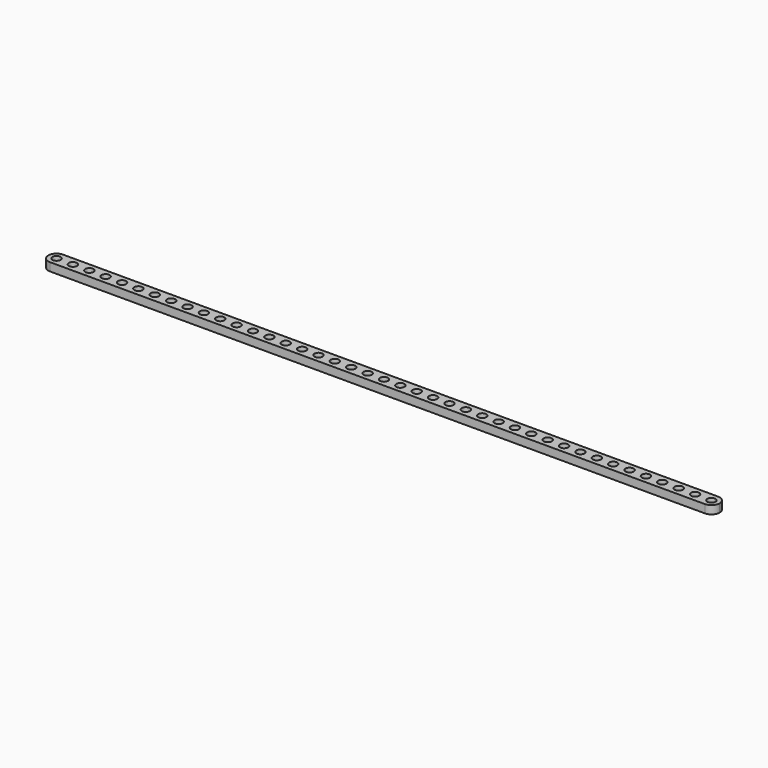
from build123d import *

# Parameters (mm, degrees)
F0_W      = 8
F0_H      = 4
F1_DEPTH  = 16
F2_DEPTH  = 24
F3_DEPTH  = 32
F4_DEPTH  = 40
F5_DEPTH  = 48
F6_DEPTH  = 56
F7_DEPTH  = 64
F8_DEPTH  = 72
F9_DEPTH  = 80
F10_DEPTH = 88
F11_DEPTH = 96
F12_DEPTH = 104
F13_DEPTH = 120
F14_DEPTH = 136
F15_DEPTH = 152
F16_DEPTH = 168
F17_DEPTH = 184
F18_DEPTH = 232
F19_DEPTH = 280
F20_DEPTH = 328
F21_R     = 2
F22_DEPTH = 12.5
F23_R     = 3.99999
F23_2_R   = 3.99999
F23_3_R   = 3.99999
F23_4_R   = 3.99999
F23_5_R   = 3.99999
F23_6_R   = 3.99999
F23_7_R   = 3.99999
F23_8_R   = 3.99999
F23_9_R   = 3.99999
F23_10_R  = 3.99999
F23_11_R  = 3.99999
F23_12_R  = 3.99999
F23_13_R  = 3.99999
F23_14_R  = 3.99999
F23_15_R  = 3.99999
F23_16_R  = 3.99999
F23_17_R  = 3.99999
F23_18_R  = 3.99999
F23_19_R  = 3.99999
F23_20_R  = 3.99999


# Not quite as in the source:
# - a fillet or chamfer is up to 0.001 mm smaller than in the source, because OpenCascade refuses the exact size


with BuildPart() as f1:
    # F0 (on Right) → F1 (new body)
    with BuildSketch(Plane.YZ):
        Rectangle(F0_W, F0_H)
    extrude(amount=F1_DEPTH)


with BuildPart() as f2:
    # F0 (on Right) → F2 (new body)
    with BuildSketch(Plane.YZ):
        Rectangle(F0_W, F0_H)
    extrude(amount=F2_DEPTH)


with BuildPart() as f3:
    # F0 (on Right) → F3 (new body)
    with BuildSketch(Plane.YZ):
        Rectangle(F0_W, F0_H)
    extrude(amount=F3_DEPTH)


with BuildPart() as f4:
    # F0 (on Right) → F4 (new body)
    with BuildSketch(Plane.YZ):
        Rectangle(F0_W, F0_H)
    extrude(amount=F4_DEPTH)


with BuildPart() as f5:
    # F0 (on Right) → F5 (new body)
    with BuildSketch(Plane.YZ):
        Rectangle(F0_W, F0_H)
    extrude(amount=F5_DEPTH)


with BuildPart() as f6:
    # F0 (on Right) → F6 (new body)
    with BuildSketch(Plane.YZ):
        Rectangle(F0_W, F0_H)
    extrude(amount=F6_DEPTH)


with BuildPart() as f7:
    # F0 (on Right) → F7 (new body)
    with BuildSketch(Plane.YZ):
        Rectangle(F0_W, F0_H)
    extrude(amount=F7_DEPTH)


with BuildPart() as f8:
    # F0 (on Right) → F8 (new body)
    with BuildSketch(Plane.YZ):
        Rectangle(F0_W, F0_H)
    extrude(amount=F8_DEPTH)


with BuildPart() as f9:
    # F0 (on Right) → F9 (new body)
    with BuildSketch(Plane.YZ):
        Rectangle(F0_W, F0_H)
    extrude(amount=F9_DEPTH)


with BuildPart() as f10:
    # F0 (on Right) → F10 (new body)
    with BuildSketch(Plane.YZ):
        Rectangle(F0_W, F0_H)
    extrude(amount=F10_DEPTH)


with BuildPart() as f11:
    # F0 (on Right) → F11 (new body)
    with BuildSketch(Plane.YZ):
        Rectangle(F0_W, F0_H)
    extrude(amount=F11_DEPTH)


with BuildPart() as f12:
    # F0 (on Right) → F12 (new body)
    with BuildSketch(Plane.YZ):
        Rectangle(F0_W, F0_H)
    extrude(amount=F12_DEPTH)


with BuildPart() as f13:
    # F0 (on Right) → F13 (new body)
    with BuildSketch(Plane.YZ):
        Rectangle(F0_W, F0_H)
    extrude(amount=F13_DEPTH)


with BuildPart() as f14:
    # F0 (on Right) → F14 (new body)
    with BuildSketch(Plane.YZ):
        Rectangle(F0_W, F0_H)
    extrude(amount=F14_DEPTH)


with BuildPart() as f15:
    # F0 (on Right) → F15 (new body)
    with BuildSketch(Plane.YZ):
        Rectangle(F0_W, F0_H)
    extrude(amount=F15_DEPTH)


with BuildPart() as f16:
    # F0 (on Right) → F16 (new body)
    with BuildSketch(Plane.YZ):
        Rectangle(F0_W, F0_H)
    extrude(amount=F16_DEPTH)


with BuildPart() as f17:
    # F0 (on Right) → F17 (new body)
    with BuildSketch(Plane.YZ):
        Rectangle(F0_W, F0_H)
    extrude(amount=F17_DEPTH)


with BuildPart() as f18:
    # F0 (on Right) → F18 (new body)
    with BuildSketch(Plane.YZ):
        Rectangle(F0_W, F0_H)
    extrude(amount=F18_DEPTH)


with BuildPart() as f19:
    # F0 (on Right) → F19 (new body)
    with BuildSketch(Plane.YZ):
        Rectangle(F0_W, F0_H)
    extrude(amount=F19_DEPTH)


with BuildPart() as f20:
    # F0 (on Right) → F20 (new body)
    with BuildSketch(Plane.YZ):
        Rectangle(F0_W, F0_H)
    extrude(amount=F20_DEPTH)


with BuildPart() as f22_tool:
    # F21 (on Top) → F22 (new body, symmetric)
    with BuildSketch(Plane.XY):
        with Locations((4, 0)):
            Circle(F21_R)
        with Locations((12, 0)):
            Circle(F21_R)
        with Locations((20, 0)):
            Circle(F21_R)
        with Locations((28, 0)):
            Circle(F21_R)
        with Locations((36, 0)):
            Circle(F21_R)
        with Locations((44, 0)):
            Circle(F21_R)
        with Locations((52, 0)):
            Circle(F21_R)
        with Locations((60, 0)):
            Circle(F21_R)
        with Locations((68, 0)):
            Circle(F21_R)
        with Locations((76, 0)):
            Circle(F21_R)
        with Locations((84, 0)):
            Circle(F21_R)
        with Locations((92, 0)):
            Circle(F21_R)
        with Locations((100, 0)):
            Circle(F21_R)
        with Locations((108, 0)):
            Circle(F21_R)
        with Locations((116, 0)):
            Circle(F21_R)
        with Locations((124, 0)):
            Circle(F21_R)
        with Locations((132, 0)):
            Circle(F21_R)
        with Locations((140, 0)):
            Circle(F21_R)
        with Locations((148, 0)):
            Circle(F21_R)
        with Locations((156, 0)):
            Circle(F21_R)
        with Locations((164, 0)):
            Circle(F21_R)
        with Locations((172, 0)):
            Circle(F21_R)
        with Locations((180, 0)):
            Circle(F21_R)
        with Locations((188, 0)):
            Circle(F21_R)
        with Locations((196, 0)):
            Circle(F21_R)
        with Locations((204, 0)):
            Circle(F21_R)
        with Locations((212, 0)):
            Circle(F21_R)
        with Locations((220, 0)):
            Circle(F21_R)
        with Locations((228, 0)):
            Circle(F21_R)
        with Locations((236, 0)):
            Circle(F21_R)
        with Locations((244, 0)):
            Circle(F21_R)
        with Locations((252, 0)):
            Circle(F21_R)
        with Locations((260, 0)):
            Circle(F21_R)
        with Locations((268, 0)):
            Circle(F21_R)
        with Locations((276, 0)):
            Circle(F21_R)
        with Locations((284, 0)):
            Circle(F21_R)
        with Locations((292, 0)):
            Circle(F21_R)
        with Locations((300, 0)):
            Circle(F21_R)
        with Locations((308, 0)):
            Circle(F21_R)
        with Locations((316, 0)):
            Circle(F21_R)
        with Locations((324, 0)):
            Circle(F21_R)
        with BuildLine():
            Line((4, 4), (0, 4))
            Line((0, 4), (0, 0))
            ThreePointArc((0, 0), (1.1715728753, 2.8284271247), (4, 4))
        make_face()
        with BuildLine():
            ThreePointArc((4, -4), (1.1715728753, -2.8284271247), (0, 0))
            Line((0, 0), (0, -4))
            Line((0, -4), (4, -4))
        make_face()
    extrude(amount=F22_DEPTH, both=True)


with BuildPart() as f1_1:
    add(f1.part)

    # F22: cut by f22_tool
    add(f22_tool.part, mode=Mode.SUBTRACT)

    # F23#20 (radius 4 in the source; OpenCascade refuses exactly that, so slightly less here)
    f23_20_edges = [f1_1.edges().sort_by_distance(p)[0] for p in [
        (16, -4, 0),
        (16, 4, 0),
    ]]
    fillet(f23_20_edges, radius=F23_20_R)


with BuildPart() as f2_1:
    add(f2.part)

    # F22: cut by f22_tool
    add(f22_tool.part, mode=Mode.SUBTRACT)

    # F23#19 (radius 4 in the source; OpenCascade refuses exactly that, so slightly less here)
    f23_19_edges = [f2_1.edges().sort_by_distance(p)[0] for p in [
        (24, -4, 0),
        (24, 4, 0),
    ]]
    fillet(f23_19_edges, radius=F23_19_R)


with BuildPart() as f3_1:
    add(f3.part)

    # F22: cut by f22_tool
    add(f22_tool.part, mode=Mode.SUBTRACT)

    # F23#18 (radius 4 in the source; OpenCascade refuses exactly that, so slightly less here)
    f23_18_edges = [f3_1.edges().sort_by_distance(p)[0] for p in [
        (32, -4, 0),
        (32, 4, 0),
    ]]
    fillet(f23_18_edges, radius=F23_18_R)


with BuildPart() as f4_1:
    add(f4.part)

    # F22: cut by f22_tool
    add(f22_tool.part, mode=Mode.SUBTRACT)

    # F23#17 (radius 4 in the source; OpenCascade refuses exactly that, so slightly less here)
    f23_17_edges = [f4_1.edges().sort_by_distance(p)[0] for p in [
        (40, -4, 0),
        (40, 4, 0),
    ]]
    fillet(f23_17_edges, radius=F23_17_R)


with BuildPart() as f5_1:
    add(f5.part)

    # F22: cut by f22_tool
    add(f22_tool.part, mode=Mode.SUBTRACT)

    # F23#16 (radius 4 in the source; OpenCascade refuses exactly that, so slightly less here)
    f23_16_edges = [f5_1.edges().sort_by_distance(p)[0] for p in [
        (48, -4, 0),
        (48, 4, 0),
    ]]
    fillet(f23_16_edges, radius=F23_16_R)


with BuildPart() as f6_1:
    add(f6.part)

    # F22: cut by f22_tool
    add(f22_tool.part, mode=Mode.SUBTRACT)

    # F23#15 (radius 4 in the source; OpenCascade refuses exactly that, so slightly less here)
    f23_15_edges = [f6_1.edges().sort_by_distance(p)[0] for p in [
        (56, -4, 0),
        (56, 4, 0),
    ]]
    fillet(f23_15_edges, radius=F23_15_R)


with BuildPart() as f7_1:
    add(f7.part)

    # F22: cut by f22_tool
    add(f22_tool.part, mode=Mode.SUBTRACT)

    # F23#14 (radius 4 in the source; OpenCascade refuses exactly that, so slightly less here)
    f23_14_edges = [f7_1.edges().sort_by_distance(p)[0] for p in [
        (64, -4, 0),
        (64, 4, 0),
    ]]
    fillet(f23_14_edges, radius=F23_14_R)


with BuildPart() as f8_1:
    add(f8.part)

    # F22: cut by f22_tool
    add(f22_tool.part, mode=Mode.SUBTRACT)

    # F23#13 (radius 4 in the source; OpenCascade refuses exactly that, so slightly less here)
    f23_13_edges = [f8_1.edges().sort_by_distance(p)[0] for p in [
        (72, -4, 0),
        (72, 4, 0),
    ]]
    fillet(f23_13_edges, radius=F23_13_R)


with BuildPart() as f9_1:
    add(f9.part)

    # F22: cut by f22_tool
    add(f22_tool.part, mode=Mode.SUBTRACT)

    # F23#12 (radius 4 in the source; OpenCascade refuses exactly that, so slightly less here)
    f23_12_edges = [f9_1.edges().sort_by_distance(p)[0] for p in [
        (80, -4, 0),
        (80, 4, 0),
    ]]
    fillet(f23_12_edges, radius=F23_12_R)


with BuildPart() as f10_1:
    add(f10.part)

    # F22: cut by f22_tool
    add(f22_tool.part, mode=Mode.SUBTRACT)

    # F23#11 (radius 4 in the source; OpenCascade refuses exactly that, so slightly less here)
    f23_11_edges = [f10_1.edges().sort_by_distance(p)[0] for p in [
        (88, -4, 0),
        (88, 4, 0),
    ]]
    fillet(f23_11_edges, radius=F23_11_R)


with BuildPart() as f11_1:
    add(f11.part)

    # F22: cut by f22_tool
    add(f22_tool.part, mode=Mode.SUBTRACT)

    # F23#10 (radius 4 in the source; OpenCascade refuses exactly that, so slightly less here)
    f23_10_edges = [f11_1.edges().sort_by_distance(p)[0] for p in [
        (96, -4, 0),
        (96, 4, 0),
    ]]
    fillet(f23_10_edges, radius=F23_10_R)


with BuildPart() as f12_1:
    add(f12.part)

    # F22: cut by f22_tool
    add(f22_tool.part, mode=Mode.SUBTRACT)

    # F23#9 (radius 4 in the source; OpenCascade refuses exactly that, so slightly less here)
    f23_9_edges = [f12_1.edges().sort_by_distance(p)[0] for p in [
        (104, -4, 0),
        (104, 4, 0),
    ]]
    fillet(f23_9_edges, radius=F23_9_R)


with BuildPart() as f13_1:
    add(f13.part)

    # F22: cut by f22_tool
    add(f22_tool.part, mode=Mode.SUBTRACT)

    # F23#8 (radius 4 in the source; OpenCascade refuses exactly that, so slightly less here)
    f23_8_edges = [f13_1.edges().sort_by_distance(p)[0] for p in [
        (120, -4, 0),
        (120, 4, 0),
    ]]
    fillet(f23_8_edges, radius=F23_8_R)


with BuildPart() as f14_1:
    add(f14.part)

    # F22: cut by f22_tool
    add(f22_tool.part, mode=Mode.SUBTRACT)

    # F23#7 (radius 4 in the source; OpenCascade refuses exactly that, so slightly less here)
    f23_7_edges = [f14_1.edges().sort_by_distance(p)[0] for p in [
        (136, -4, 0),
        (136, 4, 0),
    ]]
    fillet(f23_7_edges, radius=F23_7_R)


with BuildPart() as f15_1:
    add(f15.part)

    # F22: cut by f22_tool
    add(f22_tool.part, mode=Mode.SUBTRACT)

    # F23#6 (radius 4 in the source; OpenCascade refuses exactly that, so slightly less here)
    f23_6_edges = [f15_1.edges().sort_by_distance(p)[0] for p in [
        (152, -4, 0),
        (152, 4, 0),
    ]]
    fillet(f23_6_edges, radius=F23_6_R)


with BuildPart() as f16_1:
    add(f16.part)

    # F22: cut by f22_tool
    add(f22_tool.part, mode=Mode.SUBTRACT)

    # F23#5 (radius 4 in the source; OpenCascade refuses exactly that, so slightly less here)
    f23_5_edges = [f16_1.edges().sort_by_distance(p)[0] for p in [
        (168, -4, 0),
        (168, 4, 0),
    ]]
    fillet(f23_5_edges, radius=F23_5_R)


with BuildPart() as f17_1:
    add(f17.part)

    # F22: cut by f22_tool
    add(f22_tool.part, mode=Mode.SUBTRACT)

    # F23#4 (radius 4 in the source; OpenCascade refuses exactly that, so slightly less here)
    f23_4_edges = [f17_1.edges().sort_by_distance(p)[0] for p in [
        (184, -4, 0),
        (184, 4, 0),
    ]]
    fillet(f23_4_edges, radius=F23_4_R)


with BuildPart() as f18_1:
    add(f18.part)

    # F22: cut by f22_tool
    add(f22_tool.part, mode=Mode.SUBTRACT)

    # F23#3 (radius 4 in the source; OpenCascade refuses exactly that, so slightly less here)
    f23_3_edges = [f18_1.edges().sort_by_distance(p)[0] for p in [
        (232, -4, 0),
        (232, 4, 0),
    ]]
    fillet(f23_3_edges, radius=F23_3_R)


with BuildPart() as f19_1:
    add(f19.part)

    # F22: cut by f22_tool
    add(f22_tool.part, mode=Mode.SUBTRACT)

    # F23#2 (radius 4 in the source; OpenCascade refuses exactly that, so slightly less here)
    f23_2_edges = [f19_1.edges().sort_by_distance(p)[0] for p in [
        (280, -4, 0),
        (280, 4, 0),
    ]]
    fillet(f23_2_edges, radius=F23_2_R)


with BuildPart() as f20_1:
    add(f20.part)

    # F22: cut by f22_tool
    add(f22_tool.part, mode=Mode.SUBTRACT)

    # F23 (radius 4 in the source; OpenCascade refuses exactly that, so slightly less here)
    f23_edges = [f20_1.edges().sort_by_distance(p)[0] for p in [
        (328, -4, 0),
        (328, 4, 0),
    ]]
    fillet(f23_edges, radius=F23_R)


solid = Compound([f1_1.part, f2_1.part, f3_1.part, f4_1.part, f5_1.part, f6_1.part, f7_1.part, f8_1.part, f9_1.part, f10_1.part, f11_1.part, f12_1.part, f13_1.part, f14_1.part, f15_1.part, f16_1.part, f17_1.part, f18_1.part, f19_1.part, f20_1.part])
